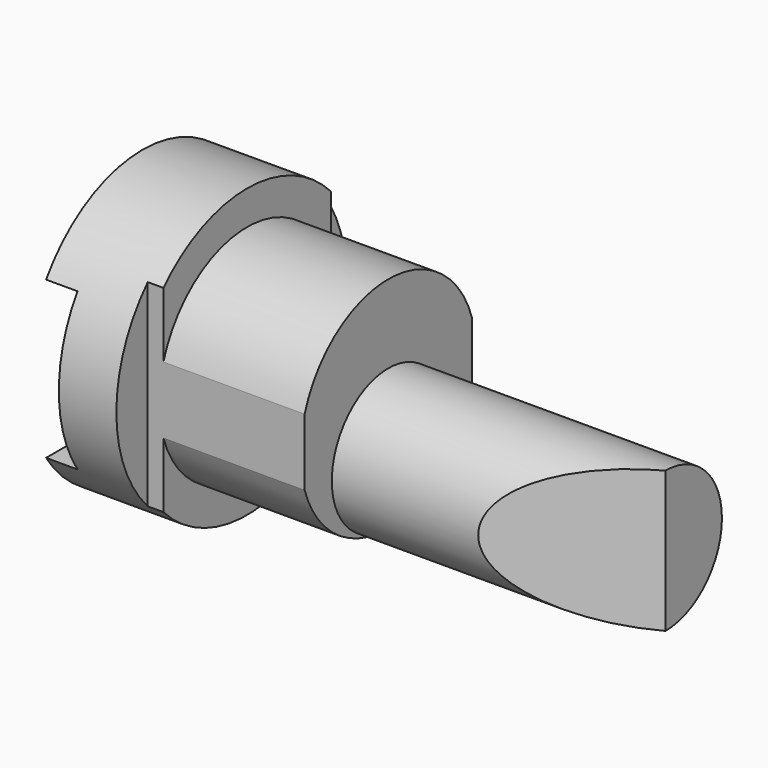
from build123d import *

# Parameters (mm, degrees)
F2_R     = 13.5
F3_DEPTH = 53
F5_DEPTH = 30
F6_W     = 6
F6_H     = 30
F7_DEPTH = 27.5
F9_DEPTH = 25


# Not quite as in the source:
# - a feature names something its author has since deleted; it is built from what else it names


with BuildPart() as f1:
    # F0 (on Front) → F1 (revolve)
    with BuildSketch(Plane.XZ):
        Polygon((0, 27.5), (0, 0), (47, 0), (47, 21), (20, 21), (20, 27.5), align=None)
    revolve(axis=Axis((37.6517102122, 0, 0), (1, 0, 0)))

    # F2 (on face) → F3 (join)
    with BuildSketch(Plane.YZ.offset(47)):
        with Locations((0, -7.5)):
            Circle(F2_R)
    extrude(amount=F3_DEPTH)

    # F4 (on face) → F5 (cut)
    with BuildSketch(Plane.YZ.offset(47)):
        with BuildLine():
            ThreePointArc((20, -18.8745860882), (25.5563103753, -10.1550480058), (27.5, 0))
            ThreePointArc((27.5, 0), (25.5563103753, 10.1550480058), (20, 18.8745860882))
            Line((20, 18.8745860882), (20, 6.4031242374))
            ThreePointArc((20, 6.4031242374), (21, 0), (20, -6.4031242374))
            Line((20, -6.4031242374), (20, -18.8745860882))
        make_face()
        with BuildLine():
            Line((-20, 6.4031242374), (-20, 18.8745860882))
            ThreePointArc((-20, 18.8745860882), (-27.5, 0), (-20, -18.8745860882))
            Line((-20, -18.8745860882), (-20, -6.4031242374))
            ThreePointArc((-20, -6.4031242374), (-21, 0), (-20, 6.4031242374))
        make_face()
        with BuildLine():
            ThreePointArc((20, -6.4031242374), (21, 0), (20, 6.4031242374))
            Line((20, 6.4031242374), (20, -6.4031242374))
        make_face()
        with BuildLine():
            Line((-20, -6.4031242374), (-20, 6.4031242374))
            ThreePointArc((-20, 6.4031242374), (-21, 0), (-20, -6.4031242374))
        make_face()
    extrude(amount=-F5_DEPTH, mode=Mode.SUBTRACT)

    # F6 (on Front) → F7 (cut, symmetric)
    with BuildSketch(Plane.XZ):
        with Locations((3, 0)):
            Rectangle(F6_W, F6_H)
    extrude(amount=F7_DEPTH, both=True, mode=Mode.SUBTRACT)

    # F8 (on Top) → F9 (cut, symmetric)
    with BuildSketch(Plane.XY):
        Polygon((100, -13.5), (100, 0), (75, -13.5), align=None)
    extrude(amount=F9_DEPTH, both=True, mode=Mode.SUBTRACT)


solid = f1.part
